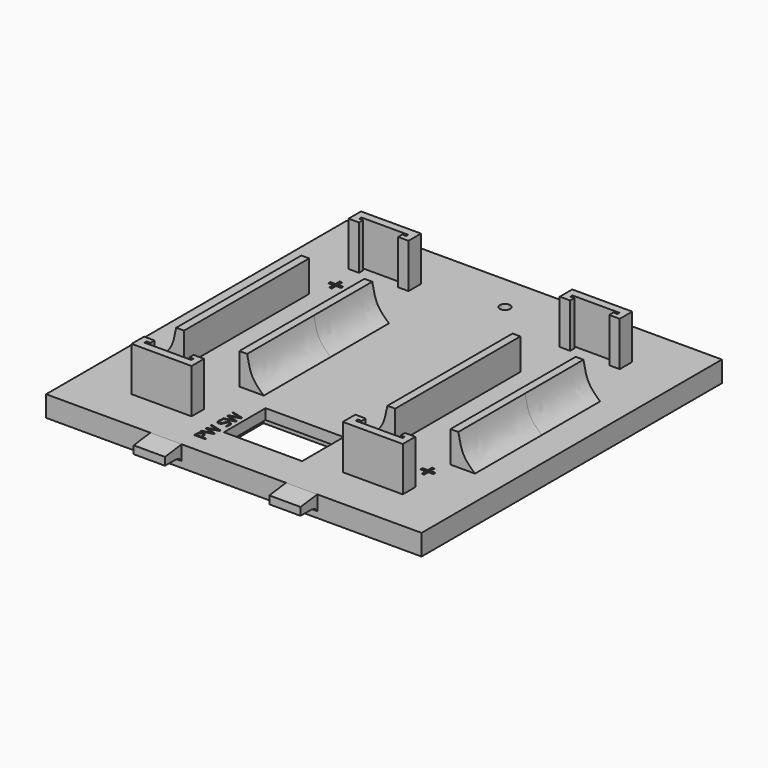
from build123d import *

# Parameters (mm, degrees)
F1_DEPTH       = 4
F2_W           = 1.5
F2_H           = 10
F3_DEPTH       = 6
F2_W_2         = 7.5
F2_H_2         = 1.5
F4_DEPTH       = 8.5
F6_R           = 1
F7_DEPTH       = 25
F8_START       = -2
F6_R_2         = 1.5
F8_DEPTH       = 23
F9_SIZE        = 1.5
F11_DEPTH      = 30
F11_DEPTH_BACK = 30
F0_W           = 20
F0_H           = 4
F12_DEPTH      = 18.6
F13_DEPTH      = 0.3
F14_W          = 15
F14_H          = 10
F15_DEPTH      = 25
F16_TEXT_SIZE  = 2.9965717759
F17_DEPTH      = 0.3
F18_R          = 4.5
F19_DEPTH      = 1
F20_W          = 19
F20_H          = 14
F21_DEPTH      = 2
F22_DEPTH      = 16
F22_DEPTH_BACK = 14


# Not quite as in the source:
# - Text() gives the source's letters only with a copy of the font that has no kerning and outlines rounded to 1/6400 em; it was checked with that copy


with BuildPart() as f1:
    # F0 (on Top) → F1 (new body)
    with BuildSketch(Plane.XY):
        Polygon((36, 36), (-36, 36), (-36, -36), (-16, -36), (-10, -36), (10, -36), (16, -36), (36, -36), align=None)
    extrude(amount=F1_DEPTH)

    # F2 (on face) → F3 (join)
    with BuildSketch(Plane.XY.offset(4)):
        with Locations((-26.3, -11)):
            Rectangle(F2_W, F2_H)
        with Locations((-14.2, -11)):
            Rectangle(F2_W, F2_H)
        with Locations((-14.2, 9)):
            Rectangle(F2_W, F2_H)
        with Locations((-26.3, 9)):
            Rectangle(F2_W, F2_H)
        with Locations((14.2, -11)):
            Rectangle(F2_W, F2_H)
        with Locations((14.2, 9)):
            Rectangle(F2_W, F2_H)
        with Locations((26.3, 9)):
            Rectangle(F2_W, F2_H)
        with Locations((26.3, -11)):
            Rectangle(F2_W, F2_H)
        with Locations((-26.3, -1)):
            Rectangle(F2_W, F2_H)
        with Locations((-14.2, -1)):
            Rectangle(F2_W, F2_H)
        with Locations((14.2, -1)):
            Rectangle(F2_W, F2_H)
        with Locations((26.3, -1)):
            Rectangle(F2_W, F2_H)
    extrude(amount=F3_DEPTH)

    # F2 (on face) → F4 (join)
    with BuildSketch(Plane.XY.offset(4)):
        Polygon((-24, 27), (-26, 27), (-26, 24), (-24, 24), (-24, 25), (-24.75, 25), (-24.75, 25.5), (-24, 25.5), align=None)
        with Locations((-20.25, 26.25)):
            Rectangle(F2_W_2, F2_H_2)
        Polygon((-14.5, 27), (-16.5, 27), (-16.5, 25.5), (-15.75, 25.5), (-15.75, 25), (-16.5, 25), (-16.5, 24), (-14.5, 24), align=None)
        Polygon((-16.5, -28), (-14.5, -28), (-14.5, -25), (-16.5, -25), (-16.5, -26), (-15.75, -26), (-15.75, -26.5), (-16.5, -26.5), align=None)
        with Locations((-20.25, -27.25)):
            Rectangle(F2_W_2, F2_H_2)
        Polygon((-26, -28), (-24, -28), (-24, -26.5), (-24.75, -26.5), (-24.75, -26), (-24, -26), (-24, -25), (-26, -25), align=None)
        Polygon((16.5, 27), (14.5, 27), (14.5, 24), (16.5, 24), (16.5, 25), (15.75, 25), (15.75, 25.5), (16.5, 25.5), align=None)
        with Locations((20.25, 26.25)):
            Rectangle(F2_W_2, F2_H_2)
        Polygon((26, 27), (24, 27), (24, 25.5), (24.75, 25.5), (24.75, 25), (24, 25), (24, 24), (26, 24), align=None)
        Polygon((24, -28), (26, -28), (26, -25), (24, -25), (24, -26), (24.75, -26), (24.75, -26.5), (24, -26.5), align=None)
        with Locations((20.25, -27.25)):
            Rectangle(F2_W_2, F2_H_2)
        Polygon((14.5, -28), (16.5, -28), (16.5, -26.5), (15.75, -26.5), (15.75, -26), (16.5, -26), (16.5, -25), (14.5, -25), align=None)
    extrude(amount=F4_DEPTH)

    # F6 (on face) → F7 (cut)
    with BuildSketch(Plane.XY.offset(4)):
        with Locations((0, 29)):
            Circle(F6_R)
    extrude(amount=-F7_DEPTH, mode=Mode.SUBTRACT)

    # F6 (on face) → F8 (cut)
    with BuildSketch(Plane.XY.offset(4).offset(F8_START)):
        with Locations((0, 29)):
            Circle(F6_R_2)
        with Locations((0, 29)):
            Circle(F6_R, mode=Mode.SUBTRACT)
    extrude(amount=-F8_DEPTH, mode=Mode.SUBTRACT)

    # F9
    f9_edges = [f1.edges().sort_by_distance(p)[0] for p in [
        (-1.5, 29, 0),
    ]]
    chamfer(f9_edges, length=F9_SIZE)

    # F10 (on Right) → F11 (join, two sides)
    with BuildSketch(Plane.YZ) as f11_sk:
        Polygon((-40, 3.5000152031), (-40, 2.0000152031), (-37.4862719295, 2.0000152031), (-36, 2.0000152031), (-36, 4.0000152031), align=None)
        with BuildLine():
            Line((-36, 2.0000152031), (-37.4862719295, 2.0000152031))
            add(Edge.make_bspline(
                [(-36, 1.1689017519), (-36.1044214362, 1.3442498086), (-36.4901854127, 1.8114031264), (-36.9847019479, 1.899799016), (-37.4862719295, 2.0000152031)],
                knots=[0, 0, 0, 0, 0.4483426834, 1, 1, 1, 1], degree=3))
            Line((-36, 1.1689017519), (-36, 2.0000152031))
        make_face()
    extrude(amount=F11_DEPTH)
    extrude(f11_sk.sketch, amount=-F11_DEPTH_BACK)

    # F0 (on Top) → F12 (cut)
    with BuildSketch(Plane.XY):
        with Locations((-26, -38)):
            Rectangle(F0_W, F0_H)
        with Locations((0, -38)):
            Rectangle(F0_W, F0_H)
        with Locations((26, -38)):
            Rectangle(F0_W, F0_H)
    extrude(amount=F12_DEPTH, mode=Mode.SUBTRACT)

    # F2 (on face) → F13 (cut)
    with BuildSketch(Plane.XY.offset(4)):
        Polygon((-24, 20), (-24.5, 20), (-24.5, 19), (-25.5, 19), (-25.5, 18.5), (-24.5, 18.5), (-24.5, 17.5), (-24, 17.5), (-24, 18.5), (-23, 18.5), (-23, 19), (-24, 19), align=None)
        Polygon((24.5, -18.5), (24, -18.5), (24, -19.5), (23, -19.5), (23, -20), (24, -20), (24, -21), (24.5, -21), (24.5, -20), (25.5, -20), (25.5, -19.5), (24.5, -19.5), align=None)
    extrude(amount=-F13_DEPTH, mode=Mode.SUBTRACT)

    # F14 (on face) → F15 (cut)
    with BuildSketch(Plane.XY.offset(4)):
        with Locations((0, -24)):
            Rectangle(F14_W, F14_H)
    extrude(amount=-F15_DEPTH, mode=Mode.SUBTRACT)

    # F16 (on face) → F17 (cut)
    with BuildSketch(Plane.XY.offset(4)):
        with Locations(Location((-8.2818013616, -32.8002534807), (0, 0, 90))):
            Text('PW SW', F16_TEXT_SIZE, font='Open Sans', text_align=(TextAlign.LEFT, TextAlign.BOTTOM))
    extrude(amount=-F17_DEPTH, mode=Mode.SUBTRACT)

    # F18 (on face) → F19 (cut)
    with BuildSketch(Plane.XY):
        with Locations((26, 26)):
            Circle(F18_R)
        with Locations((-26, 26)):
            Circle(F18_R)
        with Locations((-26, -26)):
            Circle(F18_R)
        with Locations((26, -26)):
            Circle(F18_R)
    extrude(amount=F19_DEPTH, mode=Mode.SUBTRACT)

    # F20 (on face) → F21 (cut)
    with BuildSketch(Plane(origin=(0, 0, 0), x_dir=(1, 0, 0), z_dir=(0, 0, -1))):
        with Locations((0, 24)):
            Rectangle(F20_W, F20_H)
    extrude(amount=-F21_DEPTH, mode=Mode.SUBTRACT)

    # F5 (on Front) → F22 (join, two sides)
    with BuildSketch(Plane.XZ) as f22_sk:
        with BuildLine():
            add(Edge.make_bspline(
                [(-27.05, 9.9999999995), (-27.2882756912, 8.7274690134), (-27.749279564, 6.2654397822), (-29.4304904978, 4.7379751795), (-30.2427462674, 4)],
                knots=[0, 0, 0, 0, 0.5168626652, 1, 1, 1, 1], degree=3))
            Line((-30.2427462674, 4), (-27.05, 4))
            Line((-27.05, 4), (-27.05, 9.9999999995))
        make_face()
        with BuildLine():
            add(Edge.make_bspline(
                [(-13.45, 9.9999999995), (-13.2117243088, 8.7274690134), (-12.750720436, 6.2654397822), (-11.0695095022, 4.7379751795), (-10.2572537326, 4)],
                knots=[0, 0, 0, 0, 0.5168626652, 1, 1, 1, 1], degree=3))
            Line((-13.45, 9.9999999995), (-13.45, 4))
            Line((-13.45, 4), (-10.2572537326, 4))
        make_face()
        with BuildLine():
            Line((13.45, 4), (13.45, 9.9999999995))
            add(Edge.make_bspline(
                [(13.45, 9.9999999995), (13.2117243088, 8.7274690134), (12.750720436, 6.2654397822), (11.0695095022, 4.7379751795), (10.2572537326, 4)],
                knots=[0, 0, 0, 0, 0.5168626652, 1, 1, 1, 1], degree=3))
            Line((10.2572537326, 4), (13.45, 4))
        make_face()
        with BuildLine():
            add(Edge.make_bspline(
                [(27.05, 9.9999999995), (27.2882756912, 8.7274690134), (27.749279564, 6.2654397822), (29.4304904978, 4.7379751795), (30.2427462674, 4)],
                knots=[0, 0, 0, 0, 0.5168626652, 1, 1, 1, 1], degree=3))
            Line((27.05, 9.9999999995), (27.05, 4))
            Line((27.05, 4), (30.2427462674, 4))
        make_face()
    extrude(amount=F22_DEPTH)
    extrude(f22_sk.sketch, amount=-F22_DEPTH_BACK)


solid = f1.part
